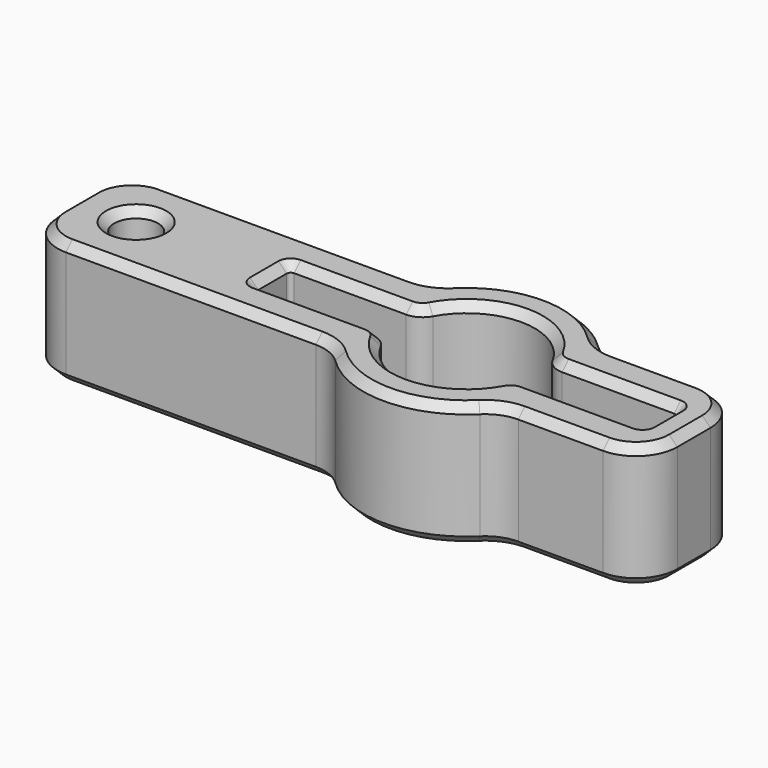
from build123d import *

# Parameters (mm, degrees)
F0_W      = 139.7
F0_H      = 38.1
F1_DEPTH  = 38.1
F2_R      = 31.75
F3_DEPTH  = 38.1
F4_W      = 119.38
F4_H      = 13.462
F5_DEPTH  = 38.101
F6_R      = 20.955
F7_DEPTH  = 38.101
F8_W      = 50.8
F8_H      = 38.1
F9_DEPTH  = 38.1
F10_R     = 12.7
F11_R     = 6.35
F12_R     = 1.27
F13_R     = 12.7
F14_R     = 6.731
F15_DEPTH = 38.101
F16_SIZE  = 2.54


with BuildPart() as f1:
    # F0 (on Top) → F1 (new body)
    with BuildSketch(Plane.XY):
        Rectangle(F0_W, F0_H)
    extrude(amount=F1_DEPTH)

    # F2 (on Top) → F3 (join, through all)
    with BuildSketch(Plane.XY):
        Circle(F2_R)
    extrude(amount=F3_DEPTH)

    # F4 (on Top) → F5 (cut, through all)
    with BuildSketch(Plane.XY):
        Rectangle(F4_W, F4_H)
    extrude(amount=F5_DEPTH, mode=Mode.SUBTRACT)

    # F6 (on Top) → F7 (cut, through all)
    with BuildSketch(Plane.XY):
        Circle(F6_R)
    extrude(amount=F7_DEPTH, mode=Mode.SUBTRACT)

    # F8 (on Top) → F9 (join, through all)
    with BuildSketch(Plane.XY):
        with Locations((-95.25, 0)):
            Rectangle(F8_W, F8_H)
    extrude(amount=F9_DEPTH)

    # F10
    f10_edges = [f1.edges().sort_by_distance(p)[0] for p in [
        (25.4, -19.05, 19.05),
        (-25.4, -19.05, 19.05),
        (25.4, 19.05, 19.05),
        (-25.4, 19.05, 19.05),
    ]]
    fillet(f10_edges, radius=F10_R)

    # F11
    f11_edges = [f1.edges().sort_by_distance(p)[0] for p in [
        (-19.844537, -6.731, 19.05),
        (19.844537, -6.731, 19.05),
        (19.844537, 6.731, 19.05),
        (-19.844537, 6.731, 19.05),
    ]]
    fillet(f11_edges, radius=F11_R)

    # F12
    f12_edges = [f1.edges().sort_by_distance(p)[0] for p in [
        (59.69, 6.731, 19.05),
        (-59.69, 6.731, 19.05),
        (-59.69, -6.731, 19.05),
        (59.69, -6.731, 19.05),
    ]]
    fillet(f12_edges, radius=F12_R)

    # F13
    f13_edges = [f1.edges().sort_by_distance(p)[0] for p in [
        (-58.42, 6.731, 19.05),
        (-58.42, -6.731, 19.05),
        (69.85, 19.05, 19.05),
        (69.85, -19.05, 19.05),
        (-120.65, -19.05, 19.05),
        (-120.65, 19.05, 19.05),
    ]]
    fillet(f13_edges, radius=F13_R)

    # F14 (on Top) → F15 (cut, through all)
    with BuildSketch(Plane.XY):
        with Locations((-101.5897616744, 0)):
            Circle(F14_R)
    extrude(amount=F15_DEPTH, mode=Mode.SUBTRACT)

    # F16
    f16_edges = [f1.edges().sort_by_distance(p)[0] for p in [
        (44.12926, 19.05, 38.1),
        (66.130256, 15.330256, 38.1),
        (26.308371, 19.992085, 38.1),
        (69.85, 0, 38.1),
        (0, 31.75, 38.1),
        (66.130256, -15.330256, 38.1),
        (-26.308371, 19.992085, 38.1),
        (44.12926, -19.05, 38.1),
        (-69.52926, 19.05, 38.1),
        (26.308371, -19.992085, 38.1),
        (-116.930256, 15.330256, 38.1),
        (0, -31.75, 38.1),
        (-120.65, 0, 38.1),
        (-26.308371, -19.992085, 38.1),
        (-116.930256, -15.330256, 38.1),
        (-69.52926, -19.05, 38.1),
        (-108.320762, 0, 38.1),
        (-41.193848, -6.731, 38.1),
        (-59.318026, -6.359026, 38.1),
        (-20.726924, -7.62024, 38.1),
        (-59.69, 0, 38.1),
        (0, -20.955, 38.1),
        (-59.318026, 6.359026, 38.1),
        (20.726924, -7.62024, 38.1),
        (-41.193848, 6.731, 38.1),
        (41.193848, -6.731, 38.1),
        (-20.726924, 7.62024, 38.1),
        (59.318026, -6.359026, 38.1),
        (0, 20.955, 38.1),
        (59.69, 0, 38.1),
        (20.726924, 7.62024, 38.1),
        (59.318026, 6.359026, 38.1),
        (41.193848, 6.731, 38.1),
        (44.12926, 19.05, 0),
        (66.130256, 15.330256, 0),
        (26.308371, 19.992085, 0),
        (69.85, 0, 0),
        (0, 31.75, 0),
        (66.130256, -15.330256, 0),
        (-26.308371, 19.992085, 0),
        (44.12926, -19.05, 0),
        (-69.52926, 19.05, 0),
        (26.308371, -19.992085, 0),
        (-116.930256, 15.330256, 0),
        (0, -31.75, 0),
        (-120.65, 0, 0),
        (-26.308371, -19.992085, 0),
        (-116.930256, -15.330256, 0),
        (-69.52926, -19.05, 0),
        (-108.320762, 0, 0),
        (41.193848, 6.731, 0),
        (59.318026, 6.359026, 0),
        (20.726924, 7.62024, 0),
        (59.69, 0, 0),
        (0, 20.955, 0),
        (59.318026, -6.359026, 0),
        (-20.726924, 7.62024, 0),
        (41.193848, -6.731, 0),
        (-41.193848, 6.731, 0),
        (20.726924, -7.62024, 0),
        (-59.318026, 6.359026, 0),
        (0, -20.955, 0),
        (-59.69, 0, 0),
        (-20.726924, -7.62024, 0),
        (-59.318026, -6.359026, 0),
        (-41.193848, -6.731, 0),
    ]]
    chamfer(f16_edges, length=F16_SIZE)


solid = f1.part
